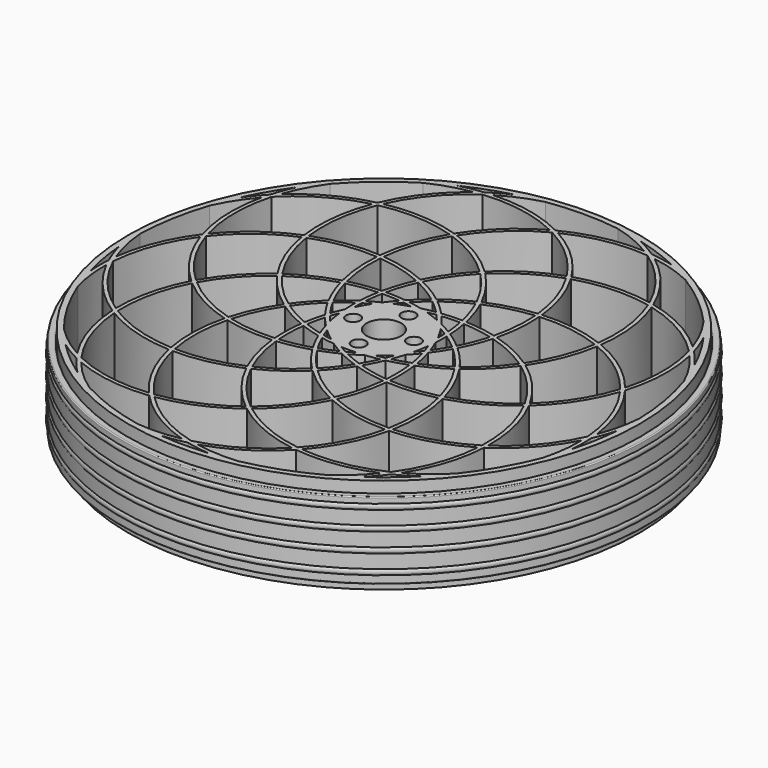
from build123d import *

# Parameters (mm, degrees)
F0_R     = 66.675
F0_R_2   = 65.175
F2_DEPTH = 12.5
F1_R     = 39.0615311231
F1_R_2   = 38.0615311231
F3_DEPTH = 12.5
F5_COUNT = 9
F6_R     = 11.2255664066
F6_R_2   = 1.8415
F6_R_3   = 4.5
F7_DEPTH = 12.5


with BuildPart() as f2:
    # F0 (on Top) → F2 (new body, symmetric)
    with BuildSketch(Plane.XY):
        Circle(F0_R)
        Circle(F0_R_2, mode=Mode.SUBTRACT)
    extrude(amount=F2_DEPTH, both=True)

    # F1 (on Top) → F3 (join, symmetric)
    with BuildSketch(Plane.XY):
        with Locations((0, 27.6134688769)):
            Circle(F1_R)
        with Locations((0, 27.6134688769)):
            Circle(F1_R_2, mode=Mode.SUBTRACT)
    extrude(amount=F3_DEPTH, both=True)


with BuildPart() as f5_1:
    # F5: instance of F2
    add(f2.part.rotate(Axis((0, 0, -0.302568078), (0, 0, -1)), 1 * 360 / F5_COUNT))


with BuildPart() as f5_2:
    # F5: instance of F2
    add(f2.part.rotate(Axis((0, 0, -0.302568078), (0, 0, -1)), 2 * 360 / F5_COUNT))


with BuildPart() as f5_3:
    # F5: instance of F2
    add(f2.part.rotate(Axis((0, 0, -0.302568078), (0, 0, -1)), 3 * 360 / F5_COUNT))


with BuildPart() as f5_4:
    # F5: instance of F2
    add(f2.part.rotate(Axis((0, 0, -0.302568078), (0, 0, -1)), 4 * 360 / F5_COUNT))


with BuildPart() as f5_5:
    # F5: instance of F2
    add(f2.part.rotate(Axis((0, 0, -0.302568078), (0, 0, -1)), 5 * 360 / F5_COUNT))


with BuildPart() as f5_6:
    # F5: instance of F2
    add(f2.part.rotate(Axis((0, 0, -0.302568078), (0, 0, -1)), 6 * 360 / F5_COUNT))


with BuildPart() as f5_7:
    # F5: instance of F2
    add(f2.part.rotate(Axis((0, 0, -0.302568078), (0, 0, -1)), 7 * 360 / F5_COUNT))


with BuildPart() as f5_8:
    # F5: instance of F2
    add(f2.part.rotate(Axis((0, 0, -0.302568078), (0, 0, -1)), 8 * 360 / F5_COUNT))


with BuildPart() as f2_1:
    add(f2.part)

    add(f5_1.part)  # F7 merges F5_1

    add(f5_2.part)  # F7 merges F5_2

    add(f5_3.part)  # F7 merges F5_3

    add(f5_4.part)  # F7 merges F5_4

    add(f5_5.part)  # F7 merges F5_5

    add(f5_6.part)  # F7 merges F5_6

    add(f5_7.part)  # F7 merges F5_7

    add(f5_8.part)  # F7 merges F5_8
    # F6 (on Top) → F7 (join, symmetric)
    with BuildSketch(Plane.XY):
        Circle(F6_R)
        with Locations((-0.1832785542, -8.0035279239)):
            Circle(F6_R_2, mode=Mode.SUBTRACT)
        with Locations((7.9101246848, -0.093403239)):
            Circle(F6_R_2, mode=Mode.SUBTRACT)
        with Locations((-8.093403239, 0.0898753152)):
            Circle(F6_R_2, mode=Mode.SUBTRACT)
        Circle(F6_R_3, mode=Mode.SUBTRACT)
        with Locations((0, 8)):
            Circle(F6_R_2, mode=Mode.SUBTRACT)
    extrude(amount=F7_DEPTH, both=True)


with BuildPart() as f9:
    # F8 (on Front) → F9 (revolve)
    with BuildSketch(Plane.XZ):
        with BuildLine():
            Line((-68.3262243271, -10.271208613), (-67.0762243271, -10.271208613))
            ThreePointArc((-67.0762243271, -10.271208613), (-66.8994476318, -10.1979853083), (-66.8262243271, -10.021208613))
            Line((-66.8262243271, -10.021208613), (-66.8262243271, -8.2283153942))
            ThreePointArc((-66.8262243271, -8.2283153942), (-67.7012243271, -8.646208613), (-68.5762243271, -8.2283153942))
            Line((-68.5762243271, -8.2283153942), (-68.5762243271, -10.021208613))
            ThreePointArc((-68.5762243271, -10.021208613), (-68.5030010224, -10.1979853083), (-68.3262243271, -10.271208613))
        make_face()
        with BuildLine():
            ThreePointArc((-68.5762243271, -8.2283153942), (-67.7012243271, -8.646208613), (-66.8262243271, -8.2283153942))
            Line((-66.8262243271, -8.2283153942), (-66.8262243271, -6.8141018318))
            ThreePointArc((-66.8262243271, -6.8141018318), (-67.7012243271, -6.396208613), (-68.5762243271, -6.8141018318))
            Line((-68.5762243271, -6.8141018318), (-68.5762243271, -8.2283153942))
        make_face()
        with BuildLine():
            Line((-66.8262243271, -6.8141018318), (-66.8262243271, -8.2283153942))
            ThreePointArc((-66.8262243271, -8.2283153942), (-66.6405641553, -7.896208613), (-66.5762243271, -7.521208613))
            ThreePointArc((-66.5762243271, -7.521208613), (-66.6405641553, -7.146208613), (-66.8262243271, -6.8141018318))
        make_face()
        with BuildLine():
            ThreePointArc((-68.5762243271, -6.8141018318), (-68.8262243271, -7.521208613), (-68.5762243271, -8.2283153942))
            Line((-68.5762243271, -8.2283153942), (-68.5762243271, -6.8141018318))
        make_face()
        with BuildLine():
            ThreePointArc((-68.5762243271, -6.8141018318), (-67.7012243271, -6.396208613), (-66.8262243271, -6.8141018318))
            Line((-66.8262243271, -6.8141018318), (-66.8262243271, -3.2283153942))
            ThreePointArc((-66.8262243271, -3.2283153942), (-67.7012243271, -3.646208613), (-68.5762243271, -3.2283153942))
            Line((-68.5762243271, -3.2283153942), (-68.5762243271, -6.8141018318))
        make_face()
        with BuildLine():
            ThreePointArc((-68.5762243271, -3.2283153942), (-67.7012243271, -3.646208613), (-66.8262243271, -3.2283153942))
            Line((-66.8262243271, -3.2283153942), (-66.8262243271, -1.8141018318))
            ThreePointArc((-66.8262243271, -1.8141018318), (-67.7012243271, -1.396208613), (-68.5762243271, -1.8141018318))
            Line((-68.5762243271, -1.8141018318), (-68.5762243271, -3.2283153942))
        make_face()
        with BuildLine():
            Line((-66.8262243271, -1.8141018318), (-66.8262243271, -3.2283153942))
            ThreePointArc((-66.8262243271, -3.2283153942), (-66.6405641553, -2.896208613), (-66.5762243271, -2.521208613))
            ThreePointArc((-66.5762243271, -2.521208613), (-66.6405641553, -2.146208613), (-66.8262243271, -1.8141018318))
        make_face()
        with BuildLine():
            ThreePointArc((-68.5762243271, -1.8141018318), (-68.8262243271, -2.521208613), (-68.5762243271, -3.2283153942))
            Line((-68.5762243271, -3.2283153942), (-68.5762243271, -1.8141018318))
        make_face()
        with BuildLine():
            ThreePointArc((-68.5762243271, -1.8141018318), (-67.7012243271, -1.396208613), (-66.8262243271, -1.8141018318))
            Line((-66.8262243271, -1.8141018318), (-66.8262243271, 1.7716846058))
            ThreePointArc((-66.8262243271, 1.7716846058), (-67.7012243271, 1.353791387), (-68.5762243271, 1.7716846058))
            Line((-68.5762243271, 1.7716846058), (-68.5762243271, -1.8141018318))
        make_face()
        with BuildLine():
            ThreePointArc((-68.5762243271, 1.7716846058), (-67.7012243271, 1.353791387), (-66.8262243271, 1.7716846058))
            Line((-66.8262243271, 1.7716846058), (-66.8262243271, 3.1858981682))
            ThreePointArc((-66.8262243271, 3.1858981682), (-67.7012243271, 3.603791387), (-68.5762243271, 3.1858981682))
            Line((-68.5762243271, 3.1858981682), (-68.5762243271, 1.7716846058))
        make_face()
        with BuildLine():
            Line((-66.8262243271, 3.1858981682), (-66.8262243271, 1.7716846058))
            ThreePointArc((-66.8262243271, 1.7716846058), (-66.6405641553, 2.103791387), (-66.5762243271, 2.478791387))
            ThreePointArc((-66.5762243271, 2.478791387), (-66.6405641553, 2.853791387), (-66.8262243271, 3.1858981682))
        make_face()
        with BuildLine():
            ThreePointArc((-68.5762243271, 3.1858981682), (-68.8262243271, 2.478791387), (-68.5762243271, 1.7716846058))
            Line((-68.5762243271, 1.7716846058), (-68.5762243271, 3.1858981682))
        make_face()
        with BuildLine():
            ThreePointArc((-68.5762243271, 3.1858981682), (-67.7012243271, 3.603791387), (-66.8262243271, 3.1858981682))
            Line((-66.8262243271, 3.1858981682), (-66.8262243271, 6.7716846058))
            ThreePointArc((-66.8262243271, 6.7716846058), (-67.7012243271, 6.353791387), (-68.5762243271, 6.7716846058))
            Line((-68.5762243271, 6.7716846058), (-68.5762243271, 3.1858981682))
        make_face()
        with BuildLine():
            ThreePointArc((-68.5762243271, 6.7716846058), (-67.7012243271, 6.353791387), (-66.8262243271, 6.7716846058))
            Line((-66.8262243271, 6.7716846058), (-66.8262243271, 8.1858981682))
            ThreePointArc((-66.8262243271, 8.1858981682), (-67.7012243271, 8.603791387), (-68.5762243271, 8.1858981682))
            Line((-68.5762243271, 8.1858981682), (-68.5762243271, 6.7716846058))
        make_face()
        with BuildLine():
            Line((-66.8262243271, 8.1858981682), (-66.8262243271, 6.7716846058))
            ThreePointArc((-66.8262243271, 6.7716846058), (-66.6405641553, 7.103791387), (-66.5762243271, 7.478791387))
            ThreePointArc((-66.5762243271, 7.478791387), (-66.6405641553, 7.853791387), (-66.8262243271, 8.1858981682))
        make_face()
        with BuildLine():
            ThreePointArc((-68.5762243271, 8.1858981682), (-68.8262243271, 7.478791387), (-68.5762243271, 6.7716846058))
            Line((-68.5762243271, 6.7716846058), (-68.5762243271, 8.1858981682))
        make_face()
        with BuildLine():
            ThreePointArc((-68.5762243271, 8.1858981682), (-67.7012243271, 8.603791387), (-66.8262243271, 8.1858981682))
            Line((-66.8262243271, 8.1858981682), (-66.8262243271, 9.478791387))
            ThreePointArc((-66.8262243271, 9.478791387), (-66.8994476318, 9.6555680823), (-67.0762243271, 9.728791387))
            Line((-67.0762243271, 9.728791387), (-68.3262243271, 9.728791387))
            ThreePointArc((-68.3262243271, 9.728791387), (-68.5030010224, 9.6555680823), (-68.5762243271, 9.478791387))
            Line((-68.5762243271, 9.478791387), (-68.5762243271, 8.1858981682))
        make_face()
    revolve(axis=Axis((0, 0, 0), (0, 0, 1)))


solid = Compound([f2_1.part, f9.part])
